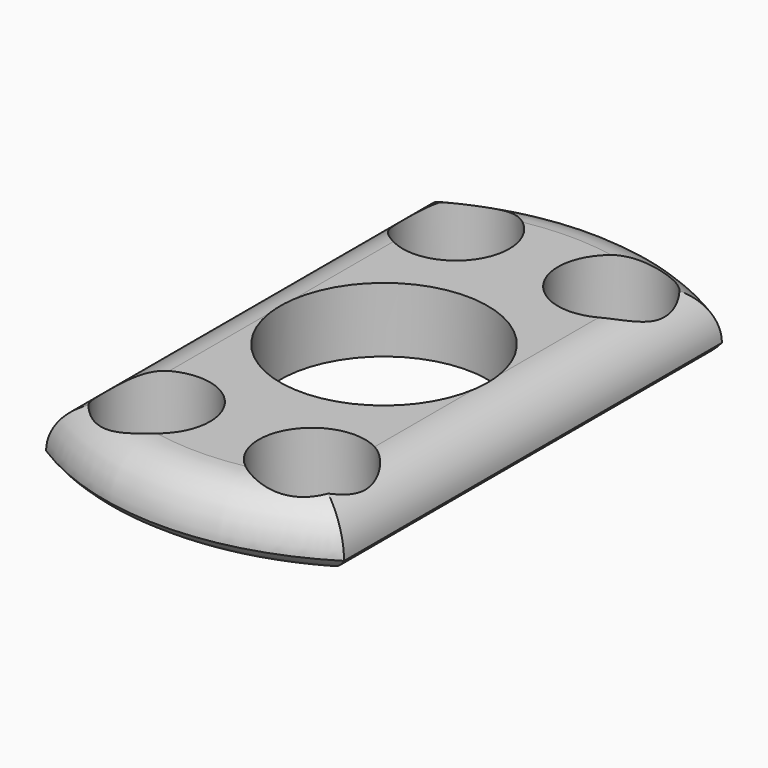
from build123d import *

# Parameters (mm, degrees)
F0_R        = 5.75
F0_R_2      = 11.2
F1_DEPTH    = 7
F2_T1_DEPTH = 76
F2_T4_ANGLE = 112.0094322503
F2_T6_ANGLE = 112.0094322503
F3_T1_DEPTH = 71.0000000002
F3_T4_ANGLE = 102.505685011
F3_T6_ANGLE = 102.505685011


# Not quite as in the source:
# - a fillet or chamfer that OpenCascade refuses, or shapes differently, is made with other operations: its cross-section is extruded or revolved along the edge and cut away or added


with BuildPart() as f1:
    # F0 (on Top) → F1 (new body)
    with BuildSketch(Plane.XY):
        with BuildLine():
            Line((16.0864073055, -25.5), (16.0864073055, 25.5))
            ThreePointArc((16.0864073055, 25.5), (0, 30.15), (-16.0864073055, 25.5))
            Line((-16.0864073055, 25.5), (-16.0864073055, -25.5))
            ThreePointArc((-16.0864073055, -25.5), (0, -30.15), (16.0864073055, -25.5))
        make_face()
        with Locations((-8.3799446002, -20.1978180557)):
            Circle(F0_R, mode=Mode.SUBTRACT)
        with Locations((8.3799446002, -20.1978180557)):
            Circle(F0_R, mode=Mode.SUBTRACT)
        with Locations((-8.3799446002, 20.1978180557)):
            Circle(F0_R, mode=Mode.SUBTRACT)
        Circle(F0_R_2, mode=Mode.SUBTRACT)
        with Locations((8.3799446002, 20.1978180557)):
            Circle(F0_R, mode=Mode.SUBTRACT)
    extrude(amount=F1_DEPTH)

    # F2: fillet of radius 5 on 4 edges, made by hand

    # F2_s2 → F2_t1 (cut)
    with BuildSketch(Plane.XZ.offset(-38)):
        with BuildLine():
            ThreePointArc((-16.0864073055, 2), (-14.6219412115, 5.5355339059), (-11.0864073055, 7))
            Line((-11.0864073055, 7), (-16.0864073055, 7))
            Line((-16.0864073055, 7), (-16.0864073055, 2))
        make_face()
        with BuildLine():
            ThreePointArc((16.0864073055, 2), (14.6219412115, 5.5355339059), (11.0864073055, 7))
            Line((11.0864073055, 7), (16.0864073055, 7))
            Line((16.0864073055, 7), (16.0864073055, 2))
        make_face()
    extrude(amount=F2_T1_DEPTH, mode=Mode.SUBTRACT)

    # F2_s3 → F2_t4 (revolve, cut)
    with BuildSketch(Plane(origin=(0, 0, 0), x_dir=(0, 0, 1), z_dir=(0.5591246619, -0.829083598, 0))):
        with BuildLine():
            ThreePointArc((2, -30.15), (5.5355339059, -28.6855339059), (7, -25.15))
            Line((7, -25.15), (7, -30.15))
            Line((7, -30.15), (2, -30.15))
        make_face()
    revolve(axis=Axis((0, 0, 7), (0, 0, 1)), revolution_arc=F2_T4_ANGLE, mode=Mode.SUBTRACT)

    # F2_s5 → F2_t6 (revolve, cut)
    with BuildSketch(Plane(origin=(0, 0, 0), x_dir=(0, 0, 1), z_dir=(-0.5591246619, 0.829083598, 0))):
        with BuildLine():
            ThreePointArc((2, -30.15), (5.5355339059, -28.6855339059), (7, -25.15))
            Line((7, -25.15), (7, -30.15))
            Line((7, -30.15), (2, -30.15))
        make_face()
    revolve(axis=Axis((0, 0, 7), (0, 0, 1)), revolution_arc=F2_T6_ANGLE, mode=Mode.SUBTRACT)

    # F3: fillet of radius 5 on 4 edges, made by hand

    # F3_s2 → F3_t1 (cut)
    with BuildSketch(Plane.XZ.offset(-35.5000000001)):
        with BuildLine():
            ThreePointArc((-12.0864073055, 0), (-14.322475283, 0.527864045), (-16.0864073055, 2))
            Line((-16.0864073055, 2), (-16.0864073055, 0))
            Line((-16.0864073055, 0), (-12.0864073055, 0))
        make_face()
        with BuildLine():
            ThreePointArc((16.0864073055, 2), (14.322475283, 0.527864045), (12.0864073055, 0))
            Line((12.0864073055, 0), (16.0864073055, 0))
            Line((16.0864073055, 0), (16.0864073055, 2))
        make_face()
    extrude(amount=F3_T1_DEPTH, mode=Mode.SUBTRACT)

    # F3_s3 → F3_t4 (revolve, cut)
    with BuildSketch(Plane(origin=(0, 0, 0), x_dir=(0, 0, 1), z_dir=(0.6258847805, -0.7799155349, 0))):
        with BuildLine():
            ThreePointArc((0, -26.15), (0.527864045, -28.3860679775), (2, -30.15))
            Line((2, -30.15), (0, -30.15))
            Line((0, -30.15), (0, -26.15))
        make_face()
    revolve(axis=Axis((0, 0, 0), (0, 0, 1)), revolution_arc=F3_T4_ANGLE, mode=Mode.SUBTRACT)

    # F3_s5 → F3_t6 (revolve, cut)
    with BuildSketch(Plane(origin=(0, 0, 0), x_dir=(0, 0, 1), z_dir=(-0.6258847805, 0.7799155349, 0))):
        with BuildLine():
            ThreePointArc((0, -26.15), (0.527864045, -28.3860679775), (2, -30.15))
            Line((2, -30.15), (0, -30.15))
            Line((0, -30.15), (0, -26.15))
        make_face()
    revolve(axis=Axis((0, 0, 0), (0, 0, 1)), revolution_arc=F3_T6_ANGLE, mode=Mode.SUBTRACT)


solid = f1.part
